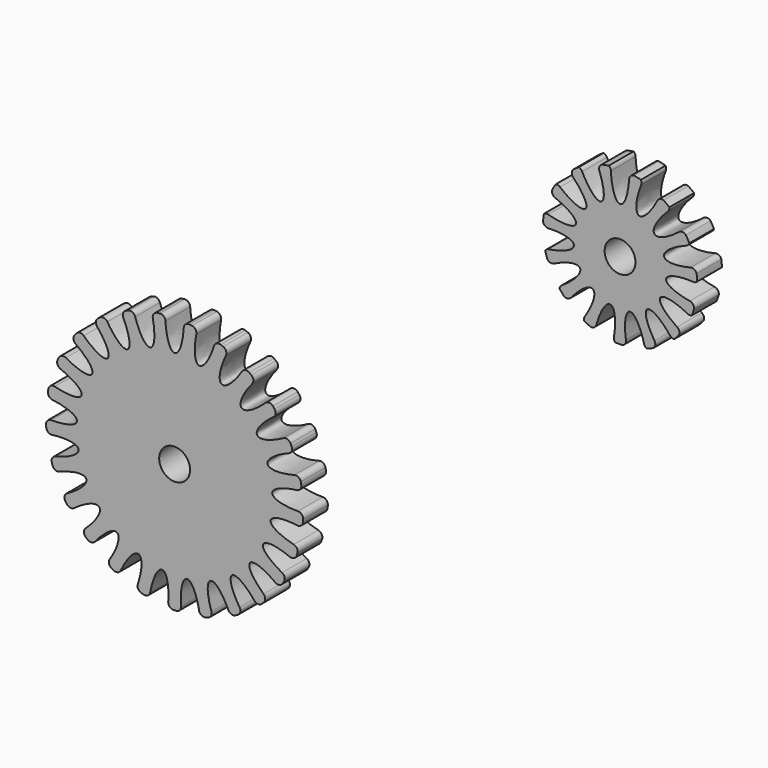
from build123d import *

# Parameters (mm, degrees)
F0_R            = 7.5
F0_R_2          = 1.5
F1_DEPTH        = 3
F0_R_3          = 12.5
F3_DEPTH        = 3.001
F3_COPIES_COUNT = 25
F5_DEPTH        = 3
F5_COPIES_COUNT = 15


# Not quite as in the source:
# - a pattern or mirror of a feature is missing from the dataset's text; its kind, count and spacing are read off the source's solid


with BuildPart() as f1:
    # F0 (on Front) → F1 (new body)
    with BuildSketch(Plane.XZ):
        with Locations((43.2630181313, 31.8110436201)):
            Circle(F0_R)
        with Locations((43.2630181313, 31.8110436201)):
            Circle(F0_R_2, mode=Mode.SUBTRACT)
    extrude(amount=F1_DEPTH)

    # F4 (on face) → F5 (cut, through all)
    with BuildSketch(Plane(origin=(0, 0, 0), x_dir=(-1, 0, 0), z_dir=(0, 1, 0))):
        with BuildLine():
            add(Edge.make_bspline(
                [(-44.1454647328, 38.719040137), (-44.0000273845, 36.3110436201), (-43.2630181313, 36.3110436201)],
                knots=[4.9110271825, 4.9110271825, 4.9110271825, 6.2831853072, 6.2831853072, 6.2831853072], degree=2, weights=[1, 0.7737359027, 1]))
            Line((-43.2630181313, 36.3110436201), (-43.2630181313, 39.3110436201))
            ThreePointArc((-43.2630181313, 39.3110436201), (-43.9421260042, 39.2802345065), (-44.6156544874, 39.1880602859))
            ThreePointArc((-44.6156544874, 39.1880602859), (-44.2914424172, 39.0428896379), (-44.1454647328, 38.719040137))
        make_face()
        with BuildLine():
            Line((-43.2630181313, 39.3110436201), (-43.2630181313, 36.3110436201))
            add(Edge.make_bspline(
                [(-43.2630181313, 36.3110436201), (-42.4904521153, 36.3110436201), (-42.3732836783, 38.8560594456)],
                knots=[0, 0, 0, 1.4185474354, 1.4185474354, 1.4185474354], degree=2, weights=[1, 0.7588350913, 1]))
            ThreePointArc((-42.3732836783, 38.8560594456), (-42.3162627291, 39.0659551169), (-42.1755168206, 39.2317808408))
            ThreePointArc((-42.1755168206, 39.2317808409), (-42.7178251175, 39.2912016785), (-43.2630181313, 39.3110436201))
        make_face()
    f5 = extrude(amount=-F5_DEPTH, mode=Mode.SUBTRACT)

    # F5_copies: F5 ×15 about axis
    f5_copies_axis = Axis((43.263018, 0, 31.811044), (0, 1, 0))
    for i in range(1, F5_COPIES_COUNT):
        add(f5.rotate(f5_copies_axis, i * 360 / F5_COPIES_COUNT), mode=Mode.SUBTRACT)


with BuildPart() as f1b:
    # F0 (on Front) → F1, piece 2 (new body)
    with BuildSketch(Plane.XZ):
        Circle(F0_R_3)
        Circle(F0_R_2, mode=Mode.SUBTRACT)
    extrude(amount=F1_DEPTH)

    # F2 (on Front) → F3 (cut, through all)
    with BuildSketch(Plane.XZ):
        with BuildLine():
            Line((0, 12.5), (0, 9.5))
            add(Edge.make_bspline(
                [(0, 9.5), (0.7471933564, 9.5), (0.8846838011, 11.9479724283)],
                knots=[0, 0, 0, 1.3857325816, 1.3857325816, 1.3857325816], degree=2, weights=[1, 0.7694183487, 1]))
            ThreePointArc((0.8846838011, 11.9479724283), (1.0619587222, 12.3024987675), (1.4415594108, 12.416598023))
            ThreePointArc((1.4415594108, 12.416598023), (0.721985011, 12.479132087), (0, 12.5))
        make_face()
        with BuildLine():
            ThreePointArc((-1.4415594108, 12.416598023), (-1.0619587222, 12.3024987675), (-0.8846838011, 11.9479724283))
            add(Edge.make_bspline(
                [(-0.8846838011, 11.9479724283), (-0.7471933564, 9.5), (0, 9.5)],
                knots=[4.8974527255, 4.8974527255, 4.8974527255, 6.2831853072, 6.2831853072, 6.2831853072], degree=2, weights=[1, 0.7694183487, 1]))
            Line((0, 9.5), (0, 12.5))
            ThreePointArc((0, 12.5), (-0.721985011, 12.479132087), (-1.4415594108, 12.416598023))
        make_face()
    f3 = extrude(amount=F3_DEPTH, mode=Mode.SUBTRACT)

    # F3_copies: F3 ×25 about axis
    f3_copies_axis = Axis((0, 0, 0), (0, 1, 0))
    for i in range(1, F3_COPIES_COUNT):
        add(f3.rotate(f3_copies_axis, i * 360 / F3_COPIES_COUNT), mode=Mode.SUBTRACT)


solid = Compound([f1.part, f1b.part])
